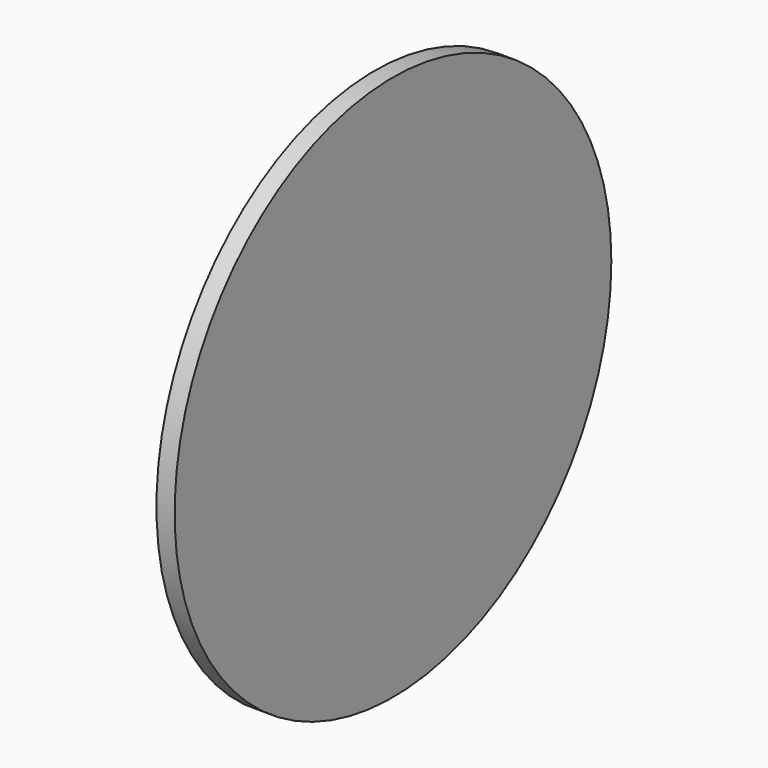
from build123d import *

# Parameters (mm, degrees)
F0_W            = 42
F0_H            = 42
F1_DEPTH        = 5
F2_R            = 1.5
F3_DEPTH        = 15
F3_COPIES_COUNT = 4
F5_R            = 45
F6_DEPTH        = 3


# Not quite as in the source:
# - a pattern or mirror of a feature is missing from the dataset's text; its kind, count and spacing are read off the source's solid


with BuildPart() as f1:
    # F0 (on Right) → F1 (new body)
    with BuildSketch(Plane.YZ):
        Rectangle(F0_W, F0_H)
    extrude(amount=F1_DEPTH)

    # F2 (on face) → F3 (cut)
    with BuildSketch(Plane.XZ.offset(21)):
        with Locations((2.5, 16)):
            Circle(F2_R)
        with Locations((2.5, 8.126)):
            Circle(F2_R)
    f3 = extrude(amount=-F3_DEPTH, mode=Mode.SUBTRACT)

    # F3_copies: F3 ×4 about axis
    f3_copies_axis = Axis((0, 0, 0), (1, 0, 0))
    for i in range(1, F3_COPIES_COUNT):
        add(f3.rotate(f3_copies_axis, i * 360 / F3_COPIES_COUNT), mode=Mode.SUBTRACT)

    # F5 (on face) → F6 (join)
    with BuildSketch(Plane.YZ.offset(5)):
        Circle(F5_R)
    extrude(amount=F6_DEPTH)


solid = f1.part
